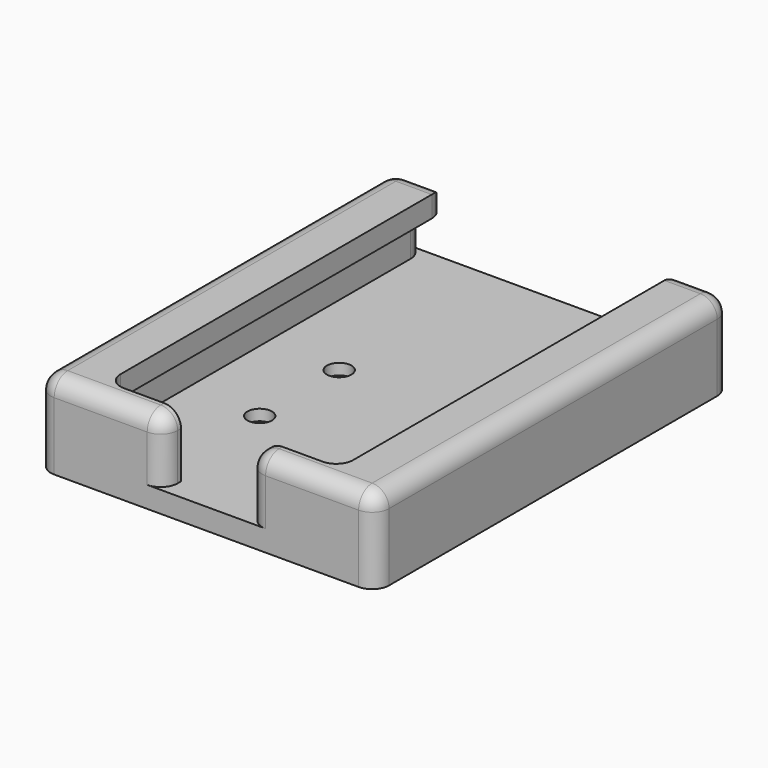
from build123d import *

# Parameters (mm, degrees)
F0_W          = 101.6
F0_H          = 127
F1_DEPTH      = 6.35
F2_W          = 9.525
F2_H          = 127
F3_DEPTH      = 12.7
F4_W          = 6.35
F4_H          = 127
F4_W_2        = 9.525
F4_W_3        = 15.875
F5_DEPTH      = 6.35
F6_R          = 3.683
F7_DEPTH      = 3.302
F8_R          = 1.9685
F9_DEPTH      = 25.4
F10_W         = 25.4
F10_H         = 6.35
F11_DEPTH     = 6.35
F12_R         = 5.08
F13_R         = 5.08
F14_T4_DEPTH  = 25.4
F14_T9_DEPTH  = 25.4
F14_T11_DEPTH = 12.7
F15_R         = 5.08


# Not quite as in the source:
# - a fillet or chamfer that OpenCascade refuses, or shapes differently, is made with other operations: its cross-section is extruded or revolved along the edge and cut away or added


with BuildPart() as f1:
    # F0 (on Top) → F1 (new body)
    with BuildSketch(Plane.XY):
        Rectangle(F0_W, F0_H)
    extrude(amount=F1_DEPTH)

    # F2 (on face) → F3 (join)
    with BuildSketch(Plane.XY.offset(6.35)):
        with Locations((-46.0375, 0)):
            Rectangle(F2_W, F2_H)
        with Locations((46.0375, 0)):
            Rectangle(F2_W, F2_H)
    extrude(amount=F3_DEPTH)

    # F4 (on face) → F5 (join)
    with BuildSketch(Plane.XY.offset(19.05)):
        with Locations((-38.1, 0)):
            Rectangle(F4_W, F4_H)
        with Locations((-46.0375, 0)):
            Rectangle(F4_W_2, F4_H)
        with Locations((42.8625, 0)):
            Rectangle(F4_W_3, F4_H)
    extrude(amount=F5_DEPTH)

    # F6 (on face) → F7 (cut)
    with BuildSketch(Plane.XY.offset(6.35)):
        with Locations((-19.05, 3.81)):
            Circle(F6_R)
        with Locations((-19.05, -26.035)):
            Circle(F6_R)
        with Locations((19.05, -26.035)):
            Circle(F6_R)
        with Locations((19.05, 3.81)):
            Circle(F6_R)
    extrude(amount=-F7_DEPTH, mode=Mode.SUBTRACT)

    # F8 (on face) → F9 (cut)
    with BuildSketch(Plane.XY.offset(3.048)):
        with Locations((-19.05, 3.81)):
            Circle(F8_R)
        with Locations((19.05, 3.81)):
            Circle(F8_R)
        with Locations((-19.05, -26.035)):
            Circle(F8_R)
        with Locations((19.05, -26.035)):
            Circle(F8_R)
    extrude(amount=-F9_DEPTH, mode=Mode.SUBTRACT)

    # F10 (on face) → F11 (join)
    with BuildSketch(Plane.XZ.offset(63.5)):
        Polygon((-34.925, 25.4), (-50.8, 25.4), (-50.8, 0), (-12.7, 0), (-12.7, 6.35), (-41.275, 6.35), (-41.275, 19.05), (-34.925, 19.05), align=None)
        Polygon((-12.7, 25.4), (-34.925, 25.4), (-34.925, 19.05), (-41.275, 19.05), (-41.275, 6.35), (-12.7, 6.35), align=None)
        Polygon((34.925, 25.4), (12.7, 25.4), (12.7, 6.35), (41.275, 6.35), (41.275, 19.05), (34.925, 19.05), align=None)
        Polygon((12.7, 6.35), (12.7, 0), (50.8, 0), (50.8, 25.4), (34.925, 25.4), (34.925, 19.05), (41.275, 19.05), (41.275, 6.35), align=None)
        with Locations((0, 3.175)):
            Rectangle(F10_W, F10_H)
    extrude(amount=F11_DEPTH)

    # F12
    f12_edges = [f1.edges().sort_by_distance(p)[0] for p in [
        (-50.8, -3.175, 25.4),
        (50.8, -3.175, 25.4),
    ]]
    fillet(f12_edges, radius=F12_R)

    # F13
    f13_edges = [f1.edges().sort_by_distance(p)[0] for p in [
        (-34.925, 63.5, 22.225),
        (34.925, 63.5, 22.225),
        (-50.8, 63.5, 10.16),
        (50.8, 63.5, 10.16),
        (-50.8, -69.85, 10.16),
        (50.8, -69.85, 10.16),
        (-34.925, -63.5, 22.225),
        (34.925, -63.5, 22.225),
    ]]
    fillet(f13_edges, radius=F13_R)

    # F14: fillet of radius 5.08 on 4 edges, made by hand


with BuildPart() as f14_tool2:
    # F14_s3 → F14_t4 (new body)
    with BuildSketch(Plane.XY.offset(6.35)):
        with BuildLine():
            ThreePointArc((-41.275, -58.42), (-39.7871024484, -62.0121024484), (-36.195, -63.5))
            Line((-36.195, -63.5), (-41.275, -63.5))
            Line((-41.275, -63.5), (-41.275, -58.42))
        make_face()
    extrude(amount=F14_T4_DEPTH)

    split(bisect_by=Plane.XY.offset(25.4), keep=Keep.BOTTOM)


with BuildPart() as f1_1:
    add(f1.part)

    # F14_t1: union F14_tool2
    add(f14_tool2.part)


with BuildPart() as f14_tool7:
    # F14_s8 → F14_t9 (new body)
    with BuildSketch(Plane.XY.offset(6.35)):
        with BuildLine():
            ThreePointArc((41.275, -58.42), (39.7871024484, -62.0121024484), (36.195, -63.5))
            Line((36.195, -63.5), (41.275, -63.5))
            Line((41.275, -63.5), (41.275, -58.42))
        make_face()
    extrude(amount=F14_T9_DEPTH)

    split(bisect_by=Plane.XY.offset(25.4), keep=Keep.BOTTOM)


with BuildPart() as f1_2:
    add(f1_1.part)

    # F14_t6: union F14_tool7
    add(f14_tool7.part)

    # F14_s12 → F14_t11 (cut)
    with BuildSketch(Plane.XY.offset(6.35)):
        with BuildLine():
            ThreePointArc((-46.355, 63.5), (-42.7628975516, 62.0121024484), (-41.275, 58.42))
            Line((-41.275, 58.42), (-41.275, 63.5))
            Line((-41.275, 63.5), (-46.355, 63.5))
        make_face()
        with BuildLine():
            ThreePointArc((46.355, 63.5), (42.7628975516, 62.0121024484), (41.275, 58.42))
            Line((41.275, 58.42), (41.275, 63.5))
            Line((41.275, 63.5), (46.355, 63.5))
        make_face()
    extrude(amount=F14_T11_DEPTH, mode=Mode.SUBTRACT)

    # F15
    f15_edges = [f1_2.edges().sort_by_distance(p)[0] for p in [
        (-12.7, -64.135, 25.4),
        (12.7, -64.135, 25.4),
        (-12.7, -69.85, 13.335),
        (12.7, -69.85, 13.335),
        (12.7, -68.362102, 23.912102),
        (-12.7, -68.362102, 23.912102),
    ]]
    fillet(f15_edges, radius=F15_R)


solid = f1_2.part
